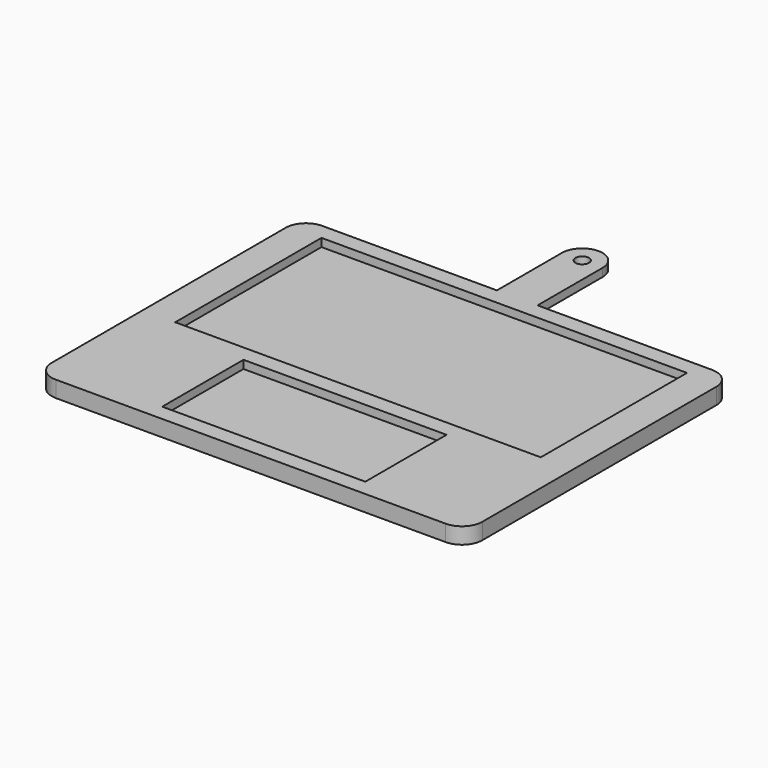
from build123d import *

# Parameters (mm, degrees)
F0_W     = 50
F0_H     = 25
F0_W_2   = 90
F0_H_2   = 45
F1_DEPTH = 4
F2_DEPTH = 2
F5_DEPTH = 2.001
F7_R     = 5
F0_R     = 1.6666666667
F8_DEPTH = 4
F9_DEPTH = 2


# Not quite as in the source:
# - a feature names something its author has since deleted; it is built from what else it names


with BuildPart() as f1:
    # F0 (on Top) → F1 (new body)
    with BuildSketch(Plane.XY):
        Polygon((-53, -84.5), (53, -84.5), (53, -2.5), (5, -2.5), (-5, -2.5), (-53, -2.5), align=None)
        with Locations((0, -68)):
            Rectangle(F0_W, F0_H, mode=Mode.SUBTRACT)
        with Locations((0, -29)):
            Rectangle(F0_W_2, F0_H_2, mode=Mode.SUBTRACT)
    extrude(amount=F1_DEPTH)

    # F0 (on Top) → F2 (join)
    with BuildSketch(Plane.XY):
        with Locations((0, -68)):
            Rectangle(F0_W, F0_H)
        with Locations((0, -29)):
            Rectangle(F0_W_2, F0_H_2)
    extrude(amount=F2_DEPTH)

    # F4 (on offset) → F5 (cut, through all)
    with BuildSketch(Plane.XY.offset(2)):
        with BuildLine():
            Line((-4.1848091993, 17.7334633669), (-4.1848091993, 13.1759698881))
            ThreePointArc((-4.1848091993, 13.1759698881), (-0.249754072, 9.1237647174), (5, 11.2082569299))
            Line((5, 11.2082569299), (5, 17.5))
            ThreePointArc((5, 17.5), (3.3860967443, 17.9195789218), (1.7383729014, 18.1759698881))
            Line((1.7383729014, 18.1759698881), (-1.7383729014, 18.1759698881))
            ThreePointArc((-1.7383729014, 18.1759698881), (-2.9698441971, 18.0003448764), (-4.1848091993, 17.7334633669))
        make_face()
        with BuildLine():
            ThreePointArc((5, 11.2082569299), (-0.249754072, 9.1237647174), (-4.1848091993, 13.1759698881))
            Line((-4.1848091993, 13.1759698881), (-4.1848091993, 17.7334633669))
            ThreePointArc((-4.1848091993, 17.7334633669), (-12.2142757372, 12.9486427976), (-16.4107558429, 4.5966133744))
            Line((-16.4107558429, 4.5966133744), (-5, -2.5))
            Line((-5, -2.5), (5, -2.5))
            Line((5, -2.5), (5, 11.2082569299))
        make_face()
    extrude(amount=-F5_DEPTH, mode=Mode.SUBTRACT)

    # F7
    f7_edges = [f1.edges().sort_by_distance(p)[0] for p in [
        (53, -84.5, 2),
        (-53, -84.5, 2),
        (-53, -2.5, 2),
        (53, -2.5, 2),
    ]]
    fillet(f7_edges, radius=F7_R)

    # F0 (on Top) → F8 (join)
    with BuildSketch(Plane.XY):
        with BuildLine():
            Line((-5, -2.5), (5, -2.5))
            Line((5, -2.5), (5, 17.5))
            ThreePointArc((5, 17.5), (0, 22.5), (-5, 17.5))
            Line((-5, 17.5), (-5, -2.5))
        make_face()
        with Locations((0, 17.5)):
            Circle(F0_R, mode=Mode.SUBTRACT)
    extrude(amount=F8_DEPTH)

    # F0 (on Top) → F9 (cut)
    with BuildSketch(Plane.XY):
        with BuildLine():
            Line((-5, -2.5), (5, -2.5))
            Line((5, -2.5), (5, 17.5))
            ThreePointArc((5, 17.5), (0, 22.5), (-5, 17.5))
            Line((-5, 17.5), (-5, -2.5))
        make_face()
        with Locations((0, 17.5)):
            Circle(F0_R, mode=Mode.SUBTRACT)
    extrude(amount=F9_DEPTH, mode=Mode.SUBTRACT)


solid = f1.part
